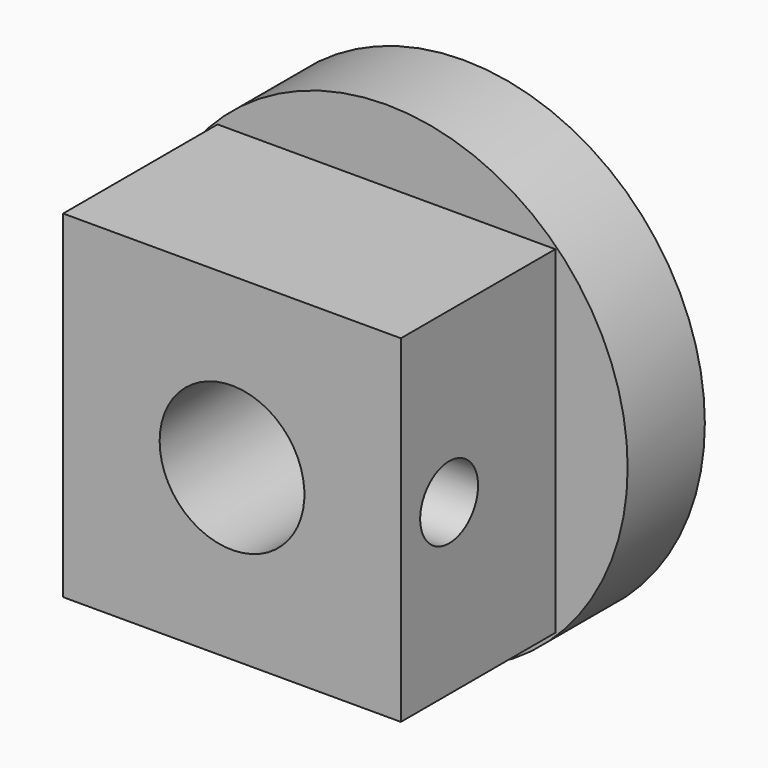
from build123d import *

# Parameters (mm, degrees)
F0_R            = 63.5
F1_DEPTH        = 25.4
F2_R            = 9.525
F3_DEPTH        = 6.35
F3_COPIES_COUNT = 8
F5_W            = 88.9
F5_H            = 88.9
F6_DEPTH        = 50.8
F4_R            = 19.05
F7_DEPTH        = 101.6
F8_R            = 9.525
F9_DEPTH        = 22.225
F10_R           = 9.525
F11_DEPTH       = 19.05


# Not quite as in the source:
# - a pattern or mirror of a feature is missing from the dataset's text; its kind, count and spacing are read off the source's solid


with BuildPart() as f1:
    # F0 (on Front) → F1 (new body)
    with BuildSketch(Plane.XZ):
        Circle(F0_R)
    extrude(amount=F1_DEPTH)

    # F2 (on face) → F3 (cut)
    with BuildSketch(Plane(origin=(0, 0, 0), x_dir=(-1, 0, 0), z_dir=(0, 1, 0))):
        with Locations((0, 50.8)):
            Circle(F2_R)
    f3 = extrude(amount=-F3_DEPTH, mode=Mode.SUBTRACT)

    # F3_copies: F3 ×8 about axis
    f3_copies_axis = Axis((0, 0, 0), (0, 1, 0))
    for i in range(1, F3_COPIES_COUNT):
        add(f3.rotate(f3_copies_axis, i * 360 / F3_COPIES_COUNT), mode=Mode.SUBTRACT)

    # F5 (on face) → F6 (join)
    with BuildSketch(Plane.XZ.offset(25.4)):
        Rectangle(F5_W, F5_H)
    extrude(amount=F6_DEPTH)

    # F4 (on face) → F7 (cut)
    with BuildSketch(Plane(origin=(0, 0, 0), x_dir=(-1, 0, 0), z_dir=(0, 1, 0))):
        Circle(F4_R)
    extrude(amount=-F7_DEPTH, mode=Mode.SUBTRACT)

    # F8 (on face) → F9 (cut)
    with BuildSketch(Plane.YZ.offset(44.45)):
        with Locations((-60.325, 0)):
            Circle(F8_R)
    extrude(amount=-F9_DEPTH, mode=Mode.SUBTRACT)

    # F10 (on face) → F11 (cut)
    with BuildSketch(Plane(origin=(-44.45, 0, 0), x_dir=(0, -1, 0), z_dir=(-1, 0, 0))):
        with Locations((60.325, 0)):
            Circle(F10_R)
    extrude(amount=-F11_DEPTH, mode=Mode.SUBTRACT)


solid = f1.part
